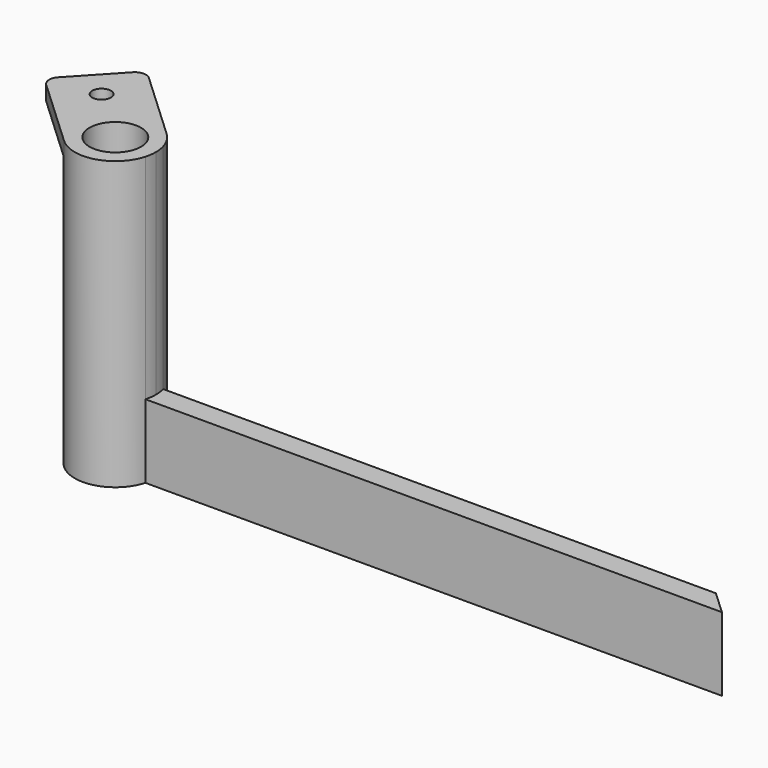
from build123d import *

# Parameters (mm, degrees)
F1_DEPTH = 10
F2_DEPTH = 39
F3_R     = 1.27
F4_DEPTH = 39
F0_R     = 1.27
F5_DEPTH = 37


# Not quite as in the source:
# - a feature names something its author has since deleted; it is built from what else it names


with BuildPart() as f1:
    # F0 (on Top) → F1 (new body)
    with BuildSketch(Plane.XY):
        with BuildLine():
            Line((35.8745669567, 1.5), (-39.2084973779, 1.5))
            ThreePointArc((-39.2084973779, 1.5), (-39.0523737086, 0.7572105316), (-39, 0))
            ThreePointArc((-39, 0), (-39.0523737086, -0.7572105316), (-39.2084973779, -1.5))
            Line((-39.2084973779, -1.5), (39.0916730868, -1.5))
            Line((39.0916730868, -1.5), (35.8745669567, 1.5))
        make_face()
    extrude(amount=F1_DEPTH)

    # F0 (on Top) → F2 (join)
    with BuildSketch(Plane.XY):
        with BuildLine():
            ThreePointArc((-46.8869942602, -2.5597379557), (-47.0597379557, 2.3869942602), (-42.1130057398, 2.5597379557))
            Line((-42.1130057398, 2.5597379557), (-40.7490090197, 4.0224453589))
            ThreePointArc((-40.7490090197, 4.0224453589), (-48.5224453589, 3.7509909803), (-48.2509909803, -4.0224453589))
            Line((-48.2509909803, -4.0224453589), (-46.8869942602, -2.5597379557))
        make_face()
        with BuildLine():
            ThreePointArc((-42.1130057398, 2.5597379557), (-41.2902897397, 1.3956217412), (-41, 0))
            ThreePointArc((-41, 0), (-43.1043782588, -3.2097102603), (-46.8869942602, -2.5597379557))
            Line((-46.8869942602, -2.5597379557), (-48.2509909803, -4.0224453589))
            ThreePointArc((-48.2509909803, -4.0224453589), (-43.0221716349, -5.2977375665), (-39.2084973779, -1.5))
            ThreePointArc((-39.2084973779, -1.5), (-39.0523737086, -0.7572105316), (-39, 0))
            ThreePointArc((-39, 0), (-39.0523737086, 0.7572105316), (-39.2084973779, 1.5))
            ThreePointArc((-39.2084973779, 1.5), (-39.8061364224, 2.866643458), (-40.7490090197, 4.0224453589))
            Line((-40.7490090197, 4.0224453589), (-42.1130057398, 2.5597379557))
        make_face()
    extrude(amount=F2_DEPTH)

    # F3 (on face) → F4 (join)
    with BuildSketch(Plane.XY):
        with BuildLine():
            Line((-57.7585891014, 4.8435333219), (-48.2509909803, -4.0224453589))
            ThreePointArc((-48.2509909803, -4.0224453589), (-48.5224453589, 3.7509909803), (-40.7490090197, 4.0224453589))
            Line((-40.7490090197, 4.0224453589), (-50.2566071407, 12.8884240397))
            ThreePointArc((-50.2566071407, 12.8884240397), (-51.3319539259, 13.2904797278), (-52.3766352332, 12.8143910274))
            Line((-52.3766352332, 12.8143910274), (-57.8326221137, 6.9635614144))
            ThreePointArc((-57.8326221137, 6.9635614144), (-58.2346778018, 5.8882146293), (-57.7585891014, 4.8435333219))
        make_face()
        with Locations((-51.8135370162, 6.8199836006)):
            Circle(F3_R, mode=Mode.SUBTRACT)
    extrude(amount=F4_DEPTH)

    # F0 (on Top) → F5 (cut)
    with BuildSketch(Plane.XY):
        with BuildLine():
            ThreePointArc((-48.2509909803, -4.0224453589), (-48.5224453589, 3.7509909803), (-40.7490090197, 4.0224453589))
            Line((-40.7490090197, 4.0224453589), (-50.2566071407, 12.8884240397))
            ThreePointArc((-50.2566071407, 12.8884240397), (-51.3319539259, 13.2904797278), (-52.3766352332, 12.8143910274))
            Line((-52.3766352332, 12.8143910274), (-57.8326221137, 6.9635614144))
            ThreePointArc((-57.8326221137, 6.9635614144), (-58.2346778018, 5.8882146293), (-57.7585891014, 4.8435333219))
            Line((-57.7585891014, 4.8435333219), (-48.2509909803, -4.0224453589))
        make_face()
        with Locations((-51.8135370162, 6.8199836006)):
            Circle(F0_R, mode=Mode.SUBTRACT)
    extrude(amount=F5_DEPTH, mode=Mode.SUBTRACT)


solid = f1.part
